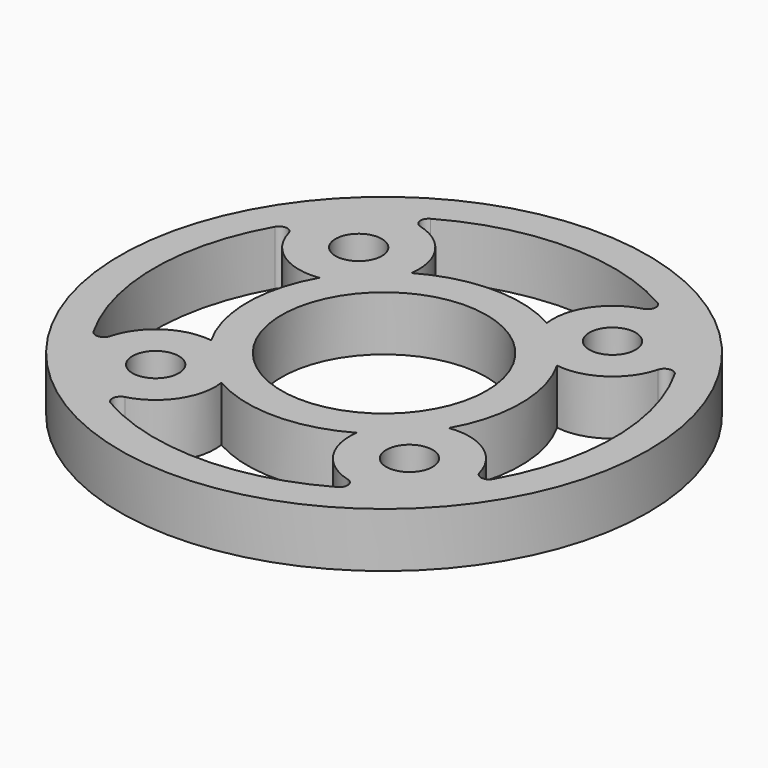
from build123d import *

# Parameters (mm, degrees)
F0_R            = 24.51608
F0_R_2          = 2.15265
F0_R_3          = 9.525
F1_DEPTH        = 5.08
F3_DEPTH        = 5.08
F3_COPIES_COUNT = 4
F4_R            = 0.762


# Not quite as in the source:
# - a pattern or mirror of a feature is missing from the dataset's text; its kind, count and spacing are read off the source's solid


with BuildPart() as f1:
    # F0 (on Top) → F1 (new body)
    with BuildSketch(Plane.XY):
        Circle(F0_R)
        with Locations((-11.7865906, -11.7865906)):
            Circle(F0_R_2, mode=Mode.SUBTRACT)
        with Locations((11.7865906, -11.7865906)):
            Circle(F0_R_2, mode=Mode.SUBTRACT)
        with Locations((-11.7865906, 11.7865906)):
            Circle(F0_R_2, mode=Mode.SUBTRACT)
        Circle(F0_R_3, mode=Mode.SUBTRACT)
        with Locations((11.7865906, 11.7865906)):
            Circle(F0_R_2, mode=Mode.SUBTRACT)
    extrude(amount=F1_DEPTH)

    # F2 (on face) → F3 (cut, through all)
    with BuildSketch(Plane.XY.offset(5.08)):
        with BuildLine():
            ThreePointArc((-12.5005198818, 17.2967828873), (-7.8454136559, 15.7030990397), (-6.2809895182, 11.0380782146))
            ThreePointArc((-6.2809895182, 11.0380782146), (0, 12.7), (6.2809895182, 11.0380782146))
            ThreePointArc((6.2809895182, 11.0380782146), (7.8454136559, 15.7030990397), (12.5005198818, 17.2967828873))
            ThreePointArc((12.5005198818, 17.2967828873), (0, 21.34108), (-12.5005198818, 17.2967828873))
        make_face()
    f3 = extrude(amount=-F3_DEPTH, mode=Mode.SUBTRACT)

    # F3_copies: F3 ×4 about axis
    f3_copies_axis = Axis((0, 0, 0), (0, 0, 1))
    for i in range(1, F3_COPIES_COUNT):
        add(f3.rotate(f3_copies_axis, i * 360 / F3_COPIES_COUNT), mode=Mode.SUBTRACT)

    # F4
    f4_edges = [f1.edges().sort_by_distance(p)[0] for p in [
        (-12.50052, 17.296783, 2.54),
        (12.50052, 17.296783, 2.54),
        (-17.296783, 12.50052, 2.54),
        (-17.296783, -12.50052, 2.54),
        (-12.50052, -17.296783, 2.54),
        (12.50052, -17.296783, 2.54),
        (17.296783, -12.50052, 2.54),
        (17.296783, 12.50052, 2.54),
    ]]
    fillet(f4_edges, radius=F4_R)


solid = f1.part
